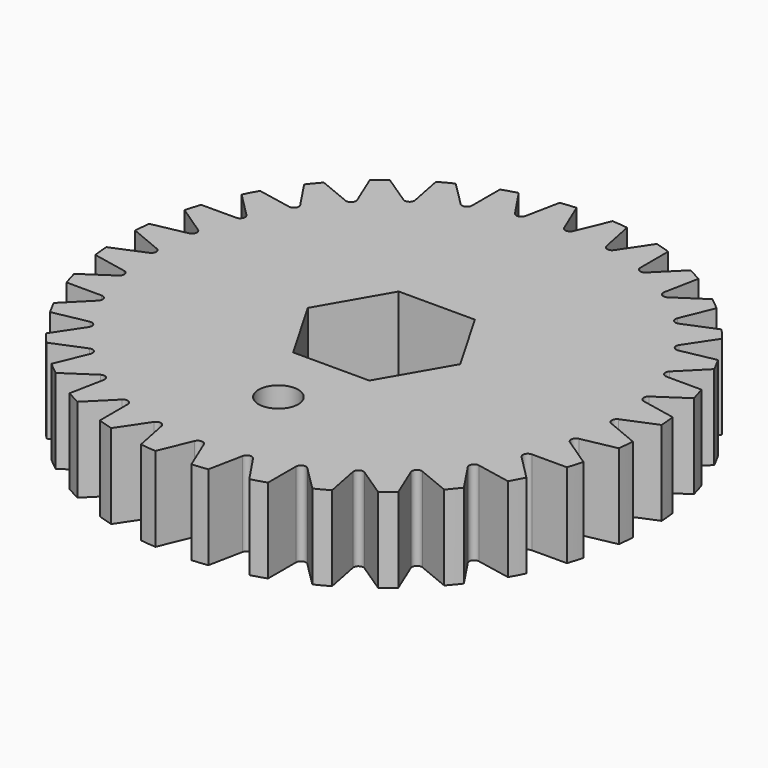
from build123d import *

# Parameters (mm, degrees)
F0_R            = 15.8688012495
F0_R_2          = 1.190625
F1_DEPTH        = 5.08
F3_DEPTH        = 5.08
F3_COPIES_COUNT = 32


# Not quite as in the source:
# - a pattern or mirror of a feature is missing from the dataset's text; its kind, count and spacing are read off the source's solid


with BuildPart() as f1:
    # F0 (on Top) → F1 (new body)
    with BuildSketch(Plane.XY):
        Circle(F0_R)
        with Locations((0, -7.9375)):
            Circle(F0_R_2, mode=Mode.SUBTRACT)
        Polygon((-4.5827177617, 0), (-2.2913588808, 3.96875), (2.2913588808, 3.96875), (4.5827177617, 0), (2.2913588808, -3.96875), (-2.2913588808, -3.96875), align=None, mode=Mode.SUBTRACT)
    extrude(amount=F1_DEPTH)

    # F2 (on face) → F3 (cut, through all)
    with BuildSketch(Plane(origin=(0, 0, 0), x_dir=(1, 0, 0), z_dir=(0, 0, -1))):
        with BuildLine():
            Line((0.2746540111, 13.8873319852), (1.0847660613, 15.8316813917))
            ThreePointArc((1.0847660613, 15.8316813917), (0, 15.8688012495), (-1.0847660613, 15.8316813917))
            Line((-1.0847660613, 15.8316813917), (-0.2746540111, 13.8873319852))
            ThreePointArc((-0.2746540111, 13.8873319852), (0, 13.7042263959), (0.2746540111, 13.8873319852))
        make_face()
    f3 = extrude(amount=-F3_DEPTH, mode=Mode.SUBTRACT)

    # F3_copies: F3 ×32 about axis
    f3_copies_axis = Axis((0, 0, 0), (0, 0, 1))
    for i in range(1, F3_COPIES_COUNT):
        add(f3.rotate(f3_copies_axis, i * 360 / F3_COPIES_COUNT), mode=Mode.SUBTRACT)


solid = f1.part
